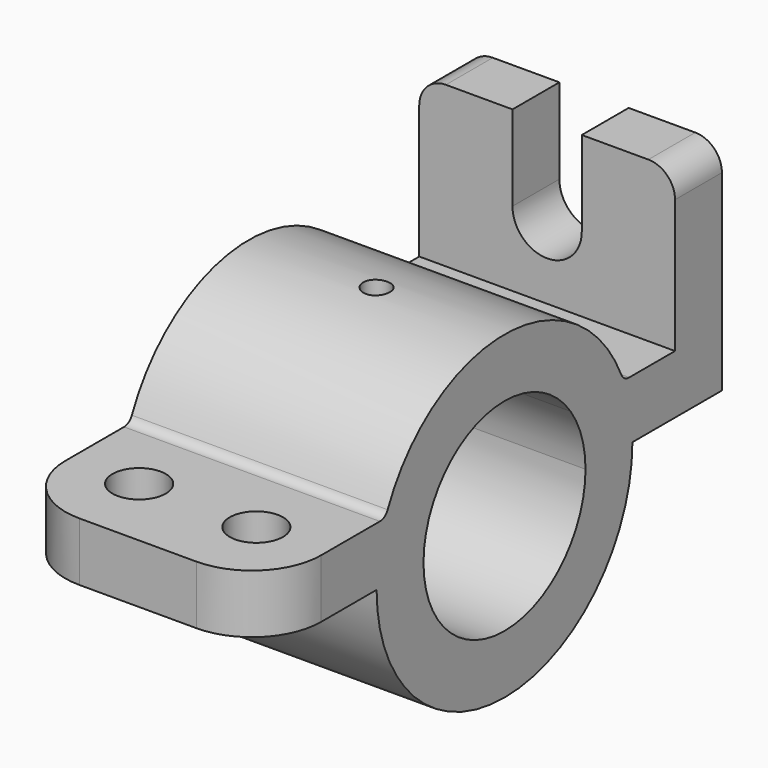
from build123d import *

# Parameters (mm, degrees)
F0_W     = 11
F0_H     = 30
F1_DEPTH = 24
F3_DEPTH = 11
F4_R     = 2.5
F4_R_2   = 5
F5_DEPTH = 41.001
F6_R     = 13
F7_R     = 5
F8_R     = 2


# Not quite as in the source:
# - a feature names something its author has since deleted; it is built from what else it names


with BuildPart() as f1:
    # F0 (on Right) → F1 (new body, symmetric)
    with BuildSketch(Plane.YZ):
        with BuildLine():
            Line((30, 0), (19, 0))
            ThreePointArc((19, 0), (0, -19), (-19, 0))
            Line((-19, 0), (-30, 0))
            ThreePointArc((-30, 0), (0, -30), (30, 0))
        make_face()
        with BuildLine():
            ThreePointArc((15.491933, 11), (18.10175, 5.772922), (19, 0))
            Line((19, 0), (30, 0))
            ThreePointArc((30, 0), (29.473014, 5.598342), (27.910571, 11))
            Line((27.910571, 11), (15.491933, 11))
        make_face()
        with BuildLine():
            ThreePointArc((-15.491933, 11), (0, 19), (15.491933, 11))
            Line((15.491933, 11), (27.910571, 11))
            ThreePointArc((27.910571, 11), (0, 30), (-27.910571, 11))
            Line((-27.910571, 11), (-15.491933, 11))
        make_face()
        with BuildLine():
            Line((-30, 0), (-19, 0))
            ThreePointArc((-19, 0), (-18.10175, 5.772922), (-15.491933, 11))
            Line((-15.491933, 11), (-27.910571, 11))
            ThreePointArc((-27.910571, 11), (-29.473014, 5.598342), (-30, 0))
        make_face()
        with BuildLine():
            ThreePointArc((27.910571, 11), (29.473014, 5.598342), (30, 0))
            Line((30, 0), (51, 0))
            Line((51, 0), (51, 11))
            Line((51, 11), (40, 11))
            Line((40, 11), (27.910571, 11))
        make_face()
        with BuildLine():
            Line((-56, 0), (-30, 0))
            ThreePointArc((-30, 0), (-29.473014, 5.598342), (-27.910571, 11))
            Line((-27.910571, 11), (-56, 11))
            Line((-56, 11), (-56, 0))
        make_face()
        with Locations((45.5, 26)):
            Rectangle(F0_W, F0_H)
    extrude(amount=F1_DEPTH, both=True)

    # F2 (on face) → F3 (cut, through all)
    with BuildSketch(Plane(origin=(0, 51, 0), x_dir=(-1, 0, 0), z_dir=(0, 1, 0))):
        with BuildLine():
            ThreePointArc((-6.5, 25), (0, 18.5), (6.5, 25))
            ThreePointArc((6.5, 25), (0, 31.5), (-6.5, 25))
        make_face()
        with BuildLine():
            ThreePointArc((-6.5, 25), (0, 31.5), (6.5, 25))
            Line((6.5, 25), (6.5, 41))
            Line((6.5, 41), (-6.5, 41))
            Line((-6.5, 41), (-6.5, 25))
        make_face()
    extrude(amount=-F3_DEPTH, mode=Mode.SUBTRACT)

    # F4 (on Top) → F5 (cut, through all)
    with BuildSketch(Plane.XY):
        Circle(F4_R)
        with Locations((-11, -41.955286)):
            Circle(F4_R_2)
        with Locations((11, -41.955286)):
            Circle(F4_R_2)
    extrude(amount=F5_DEPTH, mode=Mode.SUBTRACT)

    # F6
    f6_edges = [f1.edges().sort_by_distance(p)[0] for p in [
        (24, -56, 5.5),
        (-24, -56, 5.5),
    ]]
    fillet(f6_edges, radius=F6_R)

    # F7
    f7_edges = [f1.edges().sort_by_distance(p)[0] for p in [
        (24, 45.5, 41),
        (-24, 45.5, 41),
    ]]
    fillet(f7_edges, radius=F7_R)

    # F8
    f8_edges = [f1.edges().sort_by_distance(p)[0] for p in [
        (0, -27.910571, 11),
        (0, 27.910571, 11),
    ]]
    fillet(f8_edges, radius=F8_R)


solid = f1.part
